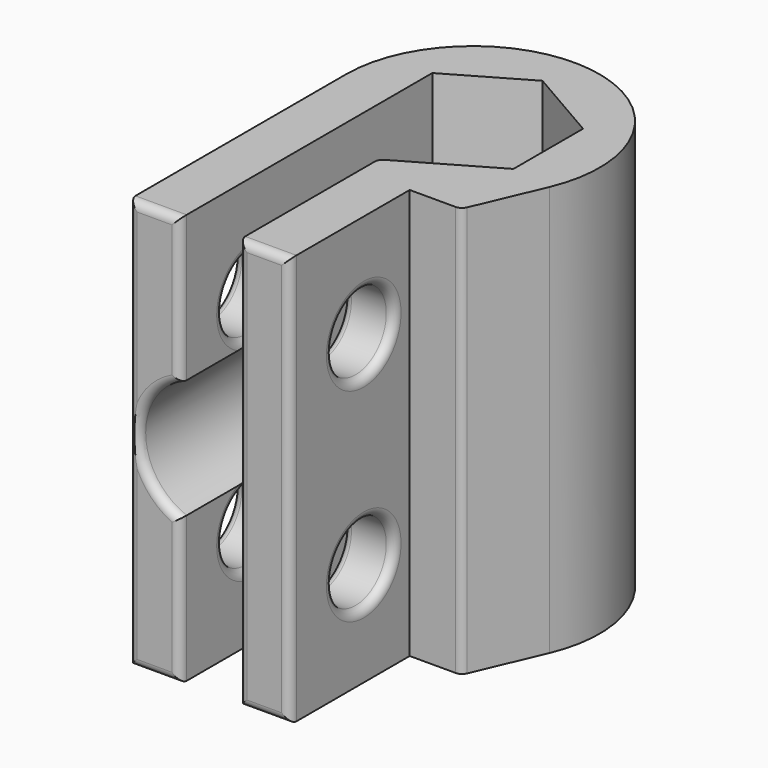
from build123d import *

# Parameters (mm, degrees)
F1_DEPTH     = 20
F2_R         = 1.875
F3_DEPTH     = 12.351
F5_DEPTH     = 7.3
F6_T1_DEPTH  = 21.1547005384
F6_T3_DEPTH  = 21.3201758156
F6_T5_DEPTH  = 22
F6_T7_DEPTH  = 4.5
F6_T9_DEPTH  = 4.5
F6_T11_DEPTH = 9.1
F6_T13_DEPTH = 9.1
F6_T32_ANGLE = 175.3394715145


# Not quite as in the source:
# - a fillet or chamfer that OpenCascade refuses, or shapes differently, is made with other operations: its cross-section is extruded or revolved along the edge and cut away or added


with BuildPart() as f1:
    # F0 (on Top) → F1 (new body)
    with BuildSketch(Plane.XY):
        with BuildLine():
            Line((-0.825, -4.7198384506), (-0.825, -6.1196405123))
            ThreePointArc((-0.825, -6.1196405123), (0.4340308681, -6.1597274457), (1.675, -5.9434838268))
            ThreePointArc((1.675, -5.9434838268), (4.0753322883, -4.6392124051), (5.6780626531, -2.4269795028))
            ThreePointArc((5.6780626531, -2.4269795028), (1.2386662418, 6.049490139), (-6.175, 0))
            ThreePointArc((-6.175, 0), (-5.5146962745, -2.7782638464), (-3.675, -4.9623583103))
            Line((-3.675, -4.9623583103), (-3.675, -2.1217622393))
            Line((-3.675, -2.1217622393), (-3.675, 0))
            Line((-3.675, 0), (-3.675, 2.1217622393))
            Line((-3.675, 2.1217622393), (0, 4.2435244785))
            Line((0, 4.2435244785), (3.675, 2.1217622393))
            Line((3.675, 2.1217622393), (3.675, -2.1217622393))
            Line((3.675, -2.1217622393), (-0.825, -4.7198384506))
        make_face()
        with BuildLine():
            ThreePointArc((1.675, -5.9434838268), (0.4340308681, -6.1597274457), (-0.825, -6.1196405123))
            Line((-0.825, -6.1196405123), (-0.825, -13.2434838268))
            Line((-0.825, -13.2434838268), (1.675, -13.2434838268))
            Line((1.675, -13.2434838268), (1.675, -5.9434838268))
        make_face()
        with BuildLine():
            ThreePointArc((5.6780626531, -2.4269795028), (4.0753322883, -4.6392124051), (1.675, -5.9434838268))
            Line((1.675, -5.9434838268), (4.175, -5.9434838268))
            Line((4.175, -5.9434838268), (5.6780626531, -2.4269795028))
        make_face()
        with BuildLine():
            ThreePointArc((-3.675, -4.9623583103), (-5.5146962745, -2.7782638464), (-6.175, 0))
            Line((-6.175, 0), (-6.175, -7.2434838268))
            Line((-6.175, -7.2434838268), (-6.175, -10.2434838268))
            Line((-6.175, -10.2434838268), (-6.175, -13.2434838268))
            Line((-6.175, -13.2434838268), (-3.675, -13.2434838268))
            Line((-3.675, -13.2434838268), (-3.675, -4.9623583103))
        make_face()
    extrude(amount=F1_DEPTH)

    # F2 (on face) → F3 (cut, through all)
    with BuildSketch(Plane(origin=(-6.175, 0, 0), x_dir=(0, -1, 0), z_dir=(-1, 0, 0))):
        with Locations((8.7434838268, 14.95)):
            Circle(F2_R)
        with Locations((8.7434838268, 5.05)):
            Circle(F2_R)
    extrude(amount=-F3_DEPTH, mode=Mode.SUBTRACT)

    # F4 (on face) → F5 (cut, through all)
    with BuildSketch(Plane.XZ.offset(13.2434838268)):
        with BuildLine():
            ThreePointArc((-3.675, 12.9), (-5.675, 10), (-3.675, 7.1))
            Line((-3.675, 7.1), (-3.675, 12.9))
        make_face()
    extrude(amount=-F5_DEPTH, mode=Mode.SUBTRACT)

    # F6: fillet of radius 0.4 on 24 edges, made by hand

    # F6_s2 → F6_t1 (cut)
    with BuildSketch(Plane.XY.offset(-0.5773502692)):
        with BuildLine():
            ThreePointArc((-0.825, -4.9507785583), (-0.7714101615, -4.7507785583), (-0.625, -4.6043683968))
            Line((-0.625, -4.6043683968), (-0.825, -4.7198384506))
            Line((-0.825, -4.7198384506), (-0.825, -4.9507785583))
        make_face()
    extrude(amount=F6_T1_DEPTH, mode=Mode.SUBTRACT)

    # F6_s4 → F6_t3 (cut)
    with BuildSketch(Plane.XY.offset(-0.6600879078)):
        with BuildLine():
            ThreePointArc((3.9109648369, -5.9434838268), (4.1313221616, -5.8773140972), (4.2787745634, -5.700697074))
            Line((4.2787745634, -5.700697074), (4.175, -5.9434838268))
            Line((4.175, -5.9434838268), (3.9109648369, -5.9434838268))
        make_face()
    extrude(amount=F6_T3_DEPTH, mode=Mode.SUBTRACT)

    # F6_s6 → F6_t5 (cut)
    with BuildSketch(Plane.XY.offset(-1)):
        with BuildLine():
            ThreePointArc((-0.825, -12.8434838268), (-0.7078427125, -13.1263265393), (-0.425, -13.2434838268))
            Line((-0.425, -13.2434838268), (-0.825, -13.2434838268))
            Line((-0.825, -13.2434838268), (-0.825, -12.8434838268))
        make_face()
        with BuildLine():
            ThreePointArc((1.275, -13.2434838268), (1.5578427125, -13.1263265393), (1.675, -12.8434838268))
            Line((1.675, -12.8434838268), (1.675, -13.2434838268))
            Line((1.675, -13.2434838268), (1.275, -13.2434838268))
        make_face()
        with BuildLine():
            ThreePointArc((-6.175, -12.8434838268), (-6.0578427125, -13.1263265393), (-5.775, -13.2434838268))
            Line((-5.775, -13.2434838268), (-6.175, -13.2434838268))
            Line((-6.175, -13.2434838268), (-6.175, -12.8434838268))
        make_face()
    extrude(amount=F6_T5_DEPTH, mode=Mode.SUBTRACT)

    # F6_s8 → F6_t7 (cut)
    with BuildSketch(Plane.YZ.offset(-1.825)):
        with BuildLine():
            ThreePointArc((-12.8434838268, 0), (-13.1263265393, 0.1171572875), (-13.2434838268, 0.4))
            Line((-13.2434838268, 0.4), (-13.2434838268, 0))
            Line((-13.2434838268, 0), (-12.8434838268, 0))
        make_face()
        with BuildLine():
            ThreePointArc((-12.8434838268, 20), (-13.1263265393, 19.8828427125), (-13.2434838268, 19.6))
            Line((-13.2434838268, 19.6), (-13.2434838268, 20))
            Line((-13.2434838268, 20), (-12.8434838268, 20))
        make_face()
    extrude(amount=F6_T7_DEPTH, mode=Mode.SUBTRACT)

    # F6_s10 → F6_t9 (cut)
    with BuildSketch(Plane.YZ.offset(-7.175)):
        with BuildLine():
            ThreePointArc((-12.8434838268, 0), (-13.1263265393, 0.1171572875), (-13.2434838268, 0.4))
            Line((-13.2434838268, 0.4), (-13.2434838268, 0))
            Line((-13.2434838268, 0), (-12.8434838268, 0))
        make_face()
        with BuildLine():
            ThreePointArc((-12.8434838268, 20), (-13.1263265393, 19.8828427125), (-13.2434838268, 19.6))
            Line((-13.2434838268, 19.6), (-13.2434838268, 20))
            Line((-13.2434838268, 20), (-12.8434838268, 20))
        make_face()
    extrude(amount=F6_T9_DEPTH, mode=Mode.SUBTRACT)

    # F6_s12 → F6_t11 (cut)
    with BuildSketch(Plane.XY.offset(-1)):
        with BuildLine():
            ThreePointArc((-4.075, -13.2434838268), (-3.7921572875, -13.1263265393), (-3.675, -12.8434838268))
            Line((-3.675, -12.8434838268), (-3.675, -13.2434838268))
            Line((-3.675, -13.2434838268), (-4.075, -13.2434838268))
        make_face()
    extrude(amount=F6_T11_DEPTH, mode=Mode.SUBTRACT)

    # F6_s14 → F6_t13 (cut)
    with BuildSketch(Plane.XY.offset(11.9)):
        with BuildLine():
            ThreePointArc((-4.075, -13.2434838268), (-3.7921572875, -13.1263265393), (-3.675, -12.8434838268))
            Line((-3.675, -12.8434838268), (-3.675, -13.2434838268))
            Line((-3.675, -13.2434838268), (-4.075, -13.2434838268))
        make_face()
    extrude(amount=F6_T13_DEPTH, mode=Mode.SUBTRACT)

    # F6_s15 → F6_t16 (revolve, cut)
    with BuildSketch(Plane.XY.offset(14.95)):
        with BuildLine():
            ThreePointArc((-0.825, -11.0184838268), (-0.7078427125, -10.7356411144), (-0.425, -10.6184838268))
            Line((-0.425, -10.6184838268), (-0.825, -10.6184838268))
            Line((-0.825, -10.6184838268), (-0.825, -11.0184838268))
        make_face()
    revolve(axis=Axis((-0.825, -8.7434838268, 14.95), (-1, 0, 0)), mode=Mode.SUBTRACT)

    # F6_s17 → F6_t18 (revolve, cut)
    with BuildSketch(Plane.XY.offset(14.95)):
        with BuildLine():
            ThreePointArc((1.275, -10.6184838268), (1.5578427125, -10.7356411144), (1.675, -11.0184838268))
            Line((1.675, -11.0184838268), (1.675, -10.6184838268))
            Line((1.675, -10.6184838268), (1.275, -10.6184838268))
        make_face()
    revolve(axis=Axis((1.675, -8.7434838268, 14.95), (-1, 0, 0)), mode=Mode.SUBTRACT)

    # F6_s19 → F6_t20 (revolve, cut)
    with BuildSketch(Plane.XY.offset(5.05)):
        with BuildLine():
            ThreePointArc((-0.825, -11.0184838268), (-0.7078427125, -10.7356411144), (-0.425, -10.6184838268))
            Line((-0.425, -10.6184838268), (-0.825, -10.6184838268))
            Line((-0.825, -10.6184838268), (-0.825, -11.0184838268))
        make_face()
    revolve(axis=Axis((-0.825, -8.7434838268, 5.05), (-1, 0, 0)), mode=Mode.SUBTRACT)

    # F6_s21 → F6_t22 (revolve, cut)
    with BuildSketch(Plane.XY.offset(5.05)):
        with BuildLine():
            ThreePointArc((1.275, -10.6184838268), (1.5578427125, -10.7356411144), (1.675, -11.0184838268))
            Line((1.675, -11.0184838268), (1.675, -10.6184838268))
            Line((1.675, -10.6184838268), (1.275, -10.6184838268))
        make_face()
    revolve(axis=Axis((1.675, -8.7434838268, 5.05), (-1, 0, 0)), mode=Mode.SUBTRACT)

    # F6_s23 → F6_t24 (revolve, cut)
    with BuildSketch(Plane.XY.offset(5.05)):
        with BuildLine():
            ThreePointArc((-6.175, -11.0184838268), (-6.0578427125, -10.7356411144), (-5.775, -10.6184838268))
            Line((-5.775, -10.6184838268), (-6.175, -10.6184838268))
            Line((-6.175, -10.6184838268), (-6.175, -11.0184838268))
        make_face()
    revolve(axis=Axis((-6.175, -8.7434838268, 5.05), (-1, 0, 0)), mode=Mode.SUBTRACT)

    # F6_s25 → F6_t26 (revolve, cut)
    with BuildSketch(Plane.XY.offset(5.05)):
        with BuildLine():
            ThreePointArc((-3.675, -11.0184838268), (-3.7921572875, -10.7356411144), (-4.075, -10.6184838268))
            Line((-4.075, -10.6184838268), (-3.675, -10.6184838268))
            Line((-3.675, -10.6184838268), (-3.675, -11.0184838268))
        make_face()
    revolve(axis=Axis((-3.675, -8.7434838268, 5.05), (-1, 0, 0)), mode=Mode.SUBTRACT)

    # F6_s27 → F6_t28 (revolve, cut)
    with BuildSketch(Plane.XY.offset(14.95)):
        with BuildLine():
            ThreePointArc((-6.175, -11.0184838268), (-6.0578427125, -10.7356411144), (-5.775, -10.6184838268))
            Line((-5.775, -10.6184838268), (-6.175, -10.6184838268))
            Line((-6.175, -10.6184838268), (-6.175, -11.0184838268))
        make_face()
    revolve(axis=Axis((-6.175, -8.7434838268, 14.95), (-1, 0, 0)), mode=Mode.SUBTRACT)

    # F6_s29 → F6_t30 (revolve, cut)
    with BuildSketch(Plane.XY.offset(14.95)):
        with BuildLine():
            ThreePointArc((-3.675, -11.0184838268), (-3.7921572875, -10.7356411144), (-4.075, -10.6184838268))
            Line((-4.075, -10.6184838268), (-3.675, -10.6184838268))
            Line((-3.675, -10.6184838268), (-3.675, -11.0184838268))
        make_face()
    revolve(axis=Axis((-3.675, -8.7434838268, 14.95), (-1, 0, 0)), mode=Mode.SUBTRACT)

    # F6_s31 → F6_t32 (revolve, cut)
    with BuildSketch(Plane(origin=(-2.1619876515, 0, -0.0879782456), x_dir=(0, 1, 0), z_dir=(0.9991730577, 0, 0.0406595721))):
        with BuildLine():
            ThreePointArc((-13.2434838268, 13.598827326), (-13.1263265393, 13.3159846135), (-12.8434838268, 13.198827326))
            Line((-12.8434838268, 13.198827326), (-13.2434838268, 13.198827326))
            Line((-13.2434838268, 13.198827326), (-13.2434838268, 13.598827326))
        make_face()
    revolve(axis=Axis((-2.5725, -13.2434838268, 10), (0, -1, 0)), revolution_arc=F6_T32_ANGLE, mode=Mode.SUBTRACT)


solid = f1.part
